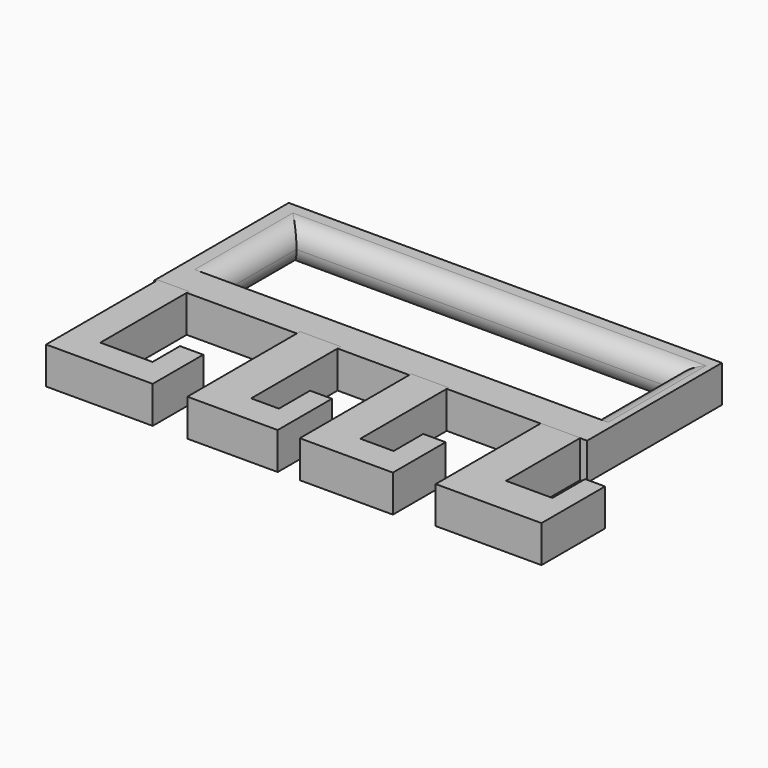
from build123d import *

# Parameters (mm, degrees)
F0_W     = 7.9836137593
F0_H     = 8.0866143107
F0_W_2   = 101.6889624298
F0_W_3   = 6.8107172847
F0_H_2   = 28.1290598214
F0_H_3   = 9.3261292204
F0_W_4   = 8.5740201175
F2_DEPTH = 10
F1_W     = 8.4114409983
F1_H     = 7.8040771186
F1_H_2   = 29.9616772681
F1_W_2   = 14.1092445701
F1_W_3   = 6.2941126525
F1_H_3   = 9.2739127576
F1_W_4   = 10.995705612
F1_H_4   = 30.2792191505
F1_W_5   = 7.4987595435
F1_W_6   = 5.9168946464
F1_H_5   = 10.5194970965
F1_W_7   = 10.1195769385
F1_H_6   = 29.8540769145
F1_W_8   = 9.0015586466
F1_W_9   = 6.0446597636
F1_H_7   = 9.9997352809
F1_W_10  = 10.6686763465
F1_H_8   = 25.1244679093
F1_H_9   = 10.4209892452
F1_W_11  = 12.5288702548
F1_W_12  = 5.3845271468
F1_H_10  = 11.0574066639
F3_R     = 4.99999


# Not quite as in the source:
# - a fillet or chamfer is up to 0.001 mm smaller than in the source, because OpenCascade refuses the exact size


with BuildPart() as f2:
    # F0 (on Top) → F2 (new body)
    with BuildSketch(Plane.XY):
        Polygon((-53.0908405781, 28.1290598214), (-53.0908405781, 36.2156741321), (-53.6812469363, 36.2156741321), (-53.6812469363, 0), (-45.1072268188, 0), (-45.1072268188, 28.1290598214), align=None)
        with Locations((-49.0990336984, 32.1723669767)):
            Rectangle(F0_W, F0_H)
        with Locations((5.7372543961, 32.1723669767)):
            Rectangle(F0_W_2, F0_H)
        with Locations((59.9870942533, 32.1723669767)):
            Rectangle(F0_W_3, F0_H)
        with Locations((59.9870942533, 14.0645299107)):
            Rectangle(F0_W_3, F0_H_2)
        with Locations((59.9870942533, -4.6630646102)):
            Rectangle(F0_W_3, F0_H_3)
        with Locations((-49.3942368776, -4.6630646102)):
            Rectangle(F0_W_4, F0_H_3)
        with Locations((5.7372543961, -4.6630646102)):
            Rectangle(F0_W_2, F0_H_3)
    extrude(amount=F2_DEPTH)

    # F3 (radius 5 in the source; OpenCascade refuses exactly that, so slightly less here)
    f3_edges = [f2.edges().sort_by_distance(p)[0] for p in [
        (-45.107227, 14.06453, 0),
        (5.737254, 28.12906, 0),
        (56.581736, 14.06453, 10),
        (5.737254, 28.12906, 10),
        (-45.107227, 14.06453, 10),
        (56.581736, 14.06453, 0),
    ]]
    fillet(f3_edges, radius=F3_R)


with BuildPart() as f2b:
    # F1 (on Top) → F2, piece 2 (new body)
    with BuildSketch(Plane.XY):
        with Locations((-49.022493884, -42.4144025892)):
            Rectangle(F1_W, F1_H)
        with Locations((-49.022493884, -23.5315253958)):
            Rectangle(F1_W, F1_H_2)
        with Locations((-37.7621510997, -42.4144025892)):
            Rectangle(F1_W_2, F1_H)
        with Locations((-27.5604724884, -42.4144025892)):
            Rectangle(F1_W_3, F1_H)
        with Locations((-27.5604724884, -33.8754076511)):
            Rectangle(F1_W_3, F1_H_3)
    extrude(amount=F2_DEPTH)


with BuildPart() as f2c:
    # F1 (on Top) → F2, piece 3 (new body)
    with BuildSketch(Plane.XY):
        with Locations((-9.5474417321, -42.4144025892)):
            Rectangle(F1_W_4, F1_H)
        with Locations((-9.5474417321, -23.3727544546)):
            Rectangle(F1_W_4, F1_H_4)
        with Locations((-0.3002091544, -42.4144025892)):
            Rectangle(F1_W_5, F1_H)
        with Locations((6.4076179406, -42.4144025892)):
            Rectangle(F1_W_6, F1_H)
        with Locations((6.4076179406, -33.2526154816)):
            Rectangle(F1_W_6, F1_H_5)
    extrude(amount=F2_DEPTH)


with BuildPart() as f2d:
    # F1 (on Top) → F2, piece 4 (new body)
    with BuildSketch(Plane.XY):
        with Locations((20.3944290988, -42.4144025892)):
            Rectangle(F1_W_7, F1_H)
        with Locations((20.3944290988, -23.5853255726)):
            Rectangle(F1_W_7, F1_H_6)
        with Locations((29.9549968913, -42.4144025892)):
            Rectangle(F1_W_8, F1_H)
        with Locations((37.4781060964, -42.4144025892)):
            Rectangle(F1_W_9, F1_H)
        with Locations((37.4781060964, -33.5124963894)):
            Rectangle(F1_W_9, F1_H_7)
    extrude(amount=F2_DEPTH)


with BuildPart() as f2e:
    # F1 (on Top) → F2, piece 5 (new body)
    with BuildSketch(Plane.XY):
        with Locations((56.1565961689, -21.7765793204)):
            Rectangle(F1_W_10, F1_H_8)
        with Locations((56.1565961689, -39.5493078977)):
            Rectangle(F1_W_10, F1_H_9)
        with Locations((67.7553694695, -39.5493078977)):
            Rectangle(F1_W_11, F1_H_9)
        with Locations((76.7120681703, -39.5493078977)):
            Rectangle(F1_W_12, F1_H_9)
        with Locations((76.7120681703, -28.8101099432)):
            Rectangle(F1_W_12, F1_H_10)
    extrude(amount=F2_DEPTH)


solid = Compound([f2.part, f2b.part, f2c.part, f2d.part, f2e.part])
